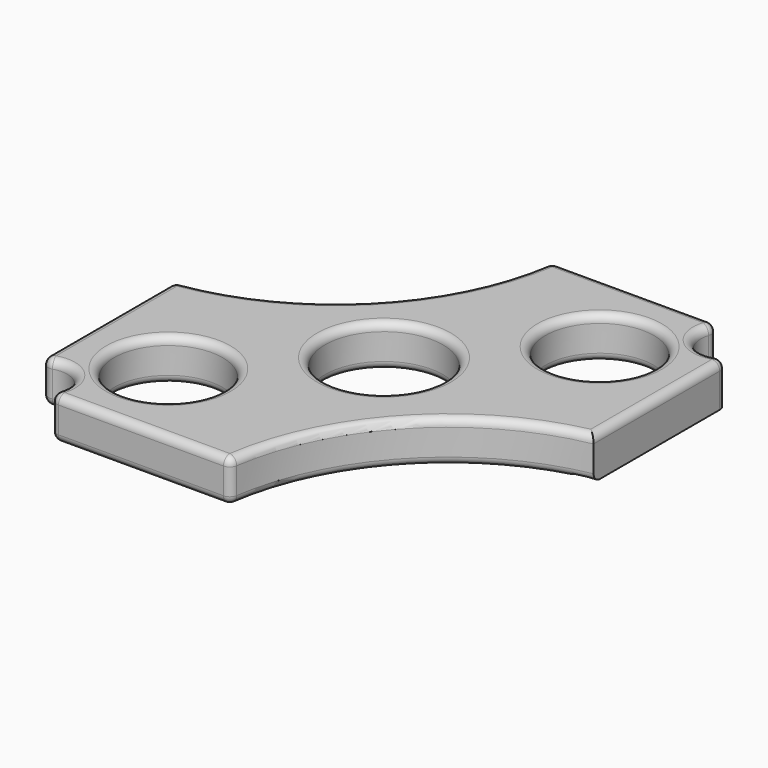
from build123d import *

# Parameters (mm, degrees)
F0_R     = 10.35
F0_R_2   = 11.25
F1_DEPTH = 8
F2_R     = 1.5


with BuildPart() as f1:
    # F0 (on Top) → F1 (new body)
    with BuildSketch(Plane.XY):
        with BuildLine():
            Line((-32.6629329423, -40.005), (2.6972468477, -40.005))
            ThreePointArc((2.6972468477, -40.005), (14.7901733739, -13.8870583483), (40, 0))
            Line((40, 0), (40, 32.6495848183))
            ThreePointArc((40, 32.6495848183), (32.8007481843, 32.8057303341), (32.6454278537, 40.005))
            Line((32.6454278537, 40.005), (0, 40.005))
            ThreePointArc((0, 40.005), (-13.1588912929, 13.1622463246), (-40, 0))
            Line((-40, 0), (-40, -32.6321214732))
            ThreePointArc((-40, -32.6321214732), (-32.8011286985, -32.805370484), (-32.6629329423, -40.005))
        make_face()
        with Locations((-22.8619287392, -22.8647864803)):
            Circle(F0_R, mode=Mode.SUBTRACT)
        Circle(F0_R_2, mode=Mode.SUBTRACT)
        with Locations((22.8676438642, 22.8590706409)):
            Circle(F0_R, mode=Mode.SUBTRACT)
    extrude(amount=F1_DEPTH)

    # F2
    f2_edges = [f1.edges().sort_by_distance(p)[0] for p in [
        (12.517644, 22.859071, 8),
        (-11.25, 0, 8),
        (-33.211929, -22.864786, 8),
        (12.517644, 22.859071, 0),
        (-11.25, 0, 0),
        (-33.211929, -22.864786, 0),
        (32.800748, 32.80573, 8),
        (40, 16.324792, 8),
        (14.790173, -13.887058, 8),
        (-14.982843, -40.005, 8),
        (-40, -16.316061, 8),
        (-32.801129, -32.80537, 8),
        (-13.158891, 13.162246, 8),
        (16.322714, 40.005, 8),
        (32.645428, 40.005, 4),
        (40, 32.649585, 4),
        (16.322714, 40.005, 0),
        (-13.158891, 13.162246, 0),
        (-40, 0, 4),
        (0, 40.005, 4),
        (-40, -16.316061, 0),
        (-40, -32.632121, 4),
        (-32.662933, -40.005, 4),
        (-32.801129, -32.80537, 0),
        (-14.982843, -40.005, 0),
        (14.790173, -13.887058, 0),
        (2.697247, -40.005, 4),
        (32.800748, 32.80573, 0),
    ]]
    fillet(f2_edges, radius=F2_R)


solid = f1.part
